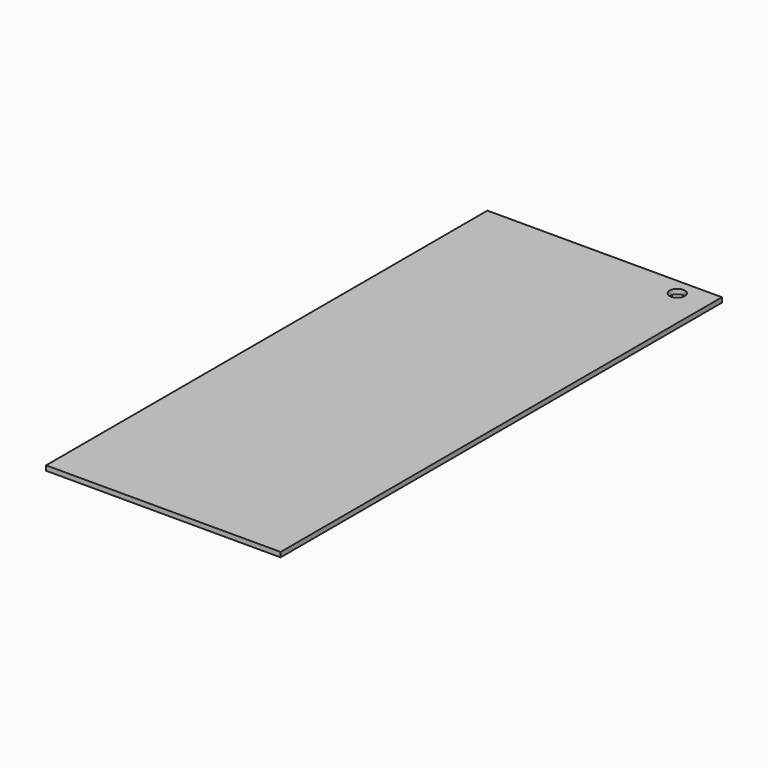
from build123d import *

# Parameters (mm, degrees)
F0_W     = 880
F0_H     = 2070
F1_DEPTH = 9
F2_R     = 28.3095234394
F3_DEPTH = 18


with BuildPart() as f1:
    # F0 (on Top) → F1 (new body, symmetric)
    with BuildSketch(Plane.XY):
        Rectangle(F0_W, F0_H)
    extrude(amount=F1_DEPTH, both=True)

    # F2 (on face) → F3 (cut)
    with BuildSketch(Plane(origin=(0, 0, -9), x_dir=(1, 0, 0), z_dir=(0, 0, -1))):
        with Locations((321.9555318356, -972.787797451)):
            Circle(F2_R)
    extrude(amount=-F3_DEPTH, mode=Mode.SUBTRACT)


solid = f1.part
